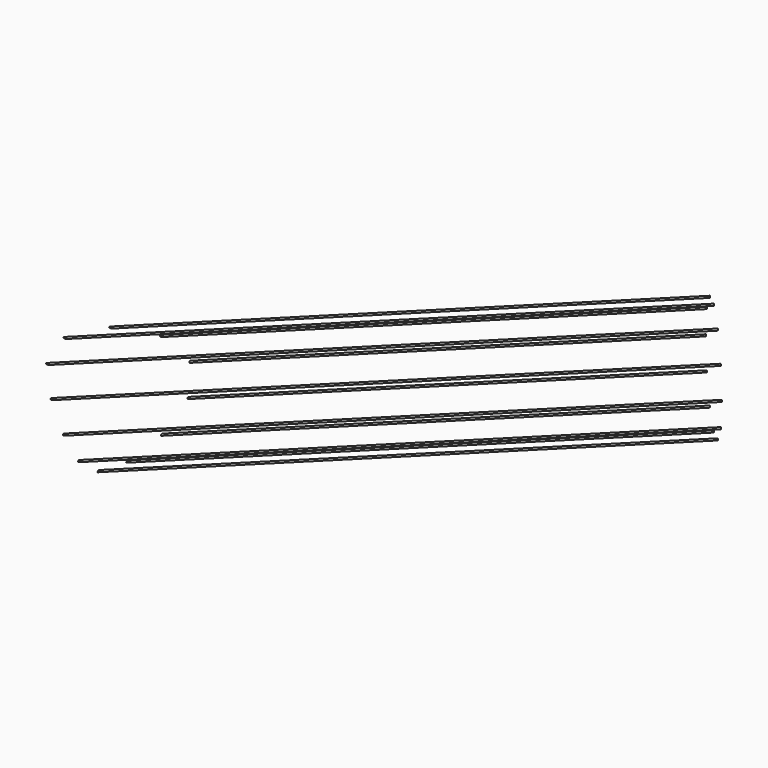
from build123d import *

# Parameters (mm, degrees)
F5_COUNT = 12
F6_R     = 101.6
F7_DEPTH = 305.3622660076


# Not quite as in the source:
# - the program builds the solid bodies; features that only make, move or delete a surface that nothing else refers to are left out


with BuildPart() as f4:
    # F3 (on offset) → F4 (revolve)
    with BuildSketch(Plane.XY.offset(25.4)):
        Polygon((0, -304.8), (0.5612660076, -305.3612660076), (431.6135598189, 125.6910278038), (431.0522938113, 126.2522938113), align=None)
    revolve(axis=Axis((215.5261469057, -89.2738530943, 25.4), (-0.7071067812, -0.7071067812, 0)))


with BuildPart() as f5_1:
    # F5: instance of F4
    add(f4.part.rotate(Axis((179.6051224214, -53.3528286101, 25.4), (0.7071067812, 0.7071067812, 0)), 1 * 360 / F5_COUNT))


with BuildPart() as f5_2:
    # F5: instance of F4
    add(f4.part.rotate(Axis((179.6051224214, -53.3528286101, 25.4), (0.7071067812, 0.7071067812, 0)), 2 * 360 / F5_COUNT))


with BuildPart() as f5_3:
    # F5: instance of F4
    add(f4.part.rotate(Axis((179.6051224214, -53.3528286101, 25.4), (0.7071067812, 0.7071067812, 0)), 3 * 360 / F5_COUNT))


with BuildPart() as f5_4:
    # F5: instance of F4
    add(f4.part.rotate(Axis((179.6051224214, -53.3528286101, 25.4), (0.7071067812, 0.7071067812, 0)), 4 * 360 / F5_COUNT))


with BuildPart() as f5_5:
    # F5: instance of F4
    add(f4.part.rotate(Axis((179.6051224214, -53.3528286101, 25.4), (0.7071067812, 0.7071067812, 0)), 5 * 360 / F5_COUNT))


with BuildPart() as f5_6:
    # F5: instance of F4
    add(f4.part.rotate(Axis((179.6051224214, -53.3528286101, 25.4), (0.7071067812, 0.7071067812, 0)), 6 * 360 / F5_COUNT))


with BuildPart() as f5_7:
    # F5: instance of F4
    add(f4.part.rotate(Axis((179.6051224214, -53.3528286101, 25.4), (0.7071067812, 0.7071067812, 0)), 7 * 360 / F5_COUNT))


with BuildPart() as f5_8:
    # F5: instance of F4
    add(f4.part.rotate(Axis((179.6051224214, -53.3528286101, 25.4), (0.7071067812, 0.7071067812, 0)), 8 * 360 / F5_COUNT))


with BuildPart() as f5_9:
    # F5: instance of F4
    add(f4.part.rotate(Axis((179.6051224214, -53.3528286101, 25.4), (0.7071067812, 0.7071067812, 0)), 9 * 360 / F5_COUNT))


with BuildPart() as f5_10:
    # F5: instance of F4
    add(f4.part.rotate(Axis((179.6051224214, -53.3528286101, 25.4), (0.7071067812, 0.7071067812, 0)), 10 * 360 / F5_COUNT))


with BuildPart() as f5_11:
    # F5: instance of F4
    add(f4.part.rotate(Axis((179.6051224214, -53.3528286101, 25.4), (0.7071067812, 0.7071067812, 0)), 11 * 360 / F5_COUNT))


with BuildPart() as f7_tool:
    # F6 (on Front) → F7 (new body, through all)
    with BuildSketch(Plane.XZ):
        Circle(F6_R)
    extrude(amount=F7_DEPTH)


with BuildPart() as f4_1:
    add(f4.part)

    # F7: cut by f7_tool
    add(f7_tool.part, mode=Mode.SUBTRACT)


with BuildPart() as f5_1_1:
    add(f5_1.part)

    # F7: cut by f7_tool
    add(f7_tool.part, mode=Mode.SUBTRACT)


with BuildPart() as f5_2_1:
    add(f5_2.part)

    # F7: cut by f7_tool
    add(f7_tool.part, mode=Mode.SUBTRACT)


with BuildPart() as f5_3_1:
    add(f5_3.part)

    # F7: cut by f7_tool
    add(f7_tool.part, mode=Mode.SUBTRACT)


with BuildPart() as f5_4_1:
    add(f5_4.part)

    # F7: cut by f7_tool
    add(f7_tool.part, mode=Mode.SUBTRACT)


with BuildPart() as f5_5_1:
    add(f5_5.part)

    # F7: cut by f7_tool
    add(f7_tool.part, mode=Mode.SUBTRACT)


with BuildPart() as f5_6_1:
    add(f5_6.part)

    # F7: cut by f7_tool
    add(f7_tool.part, mode=Mode.SUBTRACT)


with BuildPart() as f5_7_1:
    add(f5_7.part)

    # F7: cut by f7_tool
    add(f7_tool.part, mode=Mode.SUBTRACT)


with BuildPart() as f5_8_1:
    add(f5_8.part)

    # F7: cut by f7_tool
    add(f7_tool.part, mode=Mode.SUBTRACT)


with BuildPart() as f5_9_1:
    add(f5_9.part)

    # F7: cut by f7_tool
    add(f7_tool.part, mode=Mode.SUBTRACT)


with BuildPart() as f5_10_1:
    add(f5_10.part)

    # F7: cut by f7_tool
    add(f7_tool.part, mode=Mode.SUBTRACT)


with BuildPart() as f5_11_1:
    add(f5_11.part)

    # F7: cut by f7_tool
    add(f7_tool.part, mode=Mode.SUBTRACT)


solid = Compound([f4_1.part, f5_1_1.part, f5_2_1.part, f5_3_1.part, f5_4_1.part, f5_5_1.part, f5_6_1.part, f5_7_1.part, f5_8_1.part, f5_9_1.part, f5_10_1.part, f5_11_1.part])
